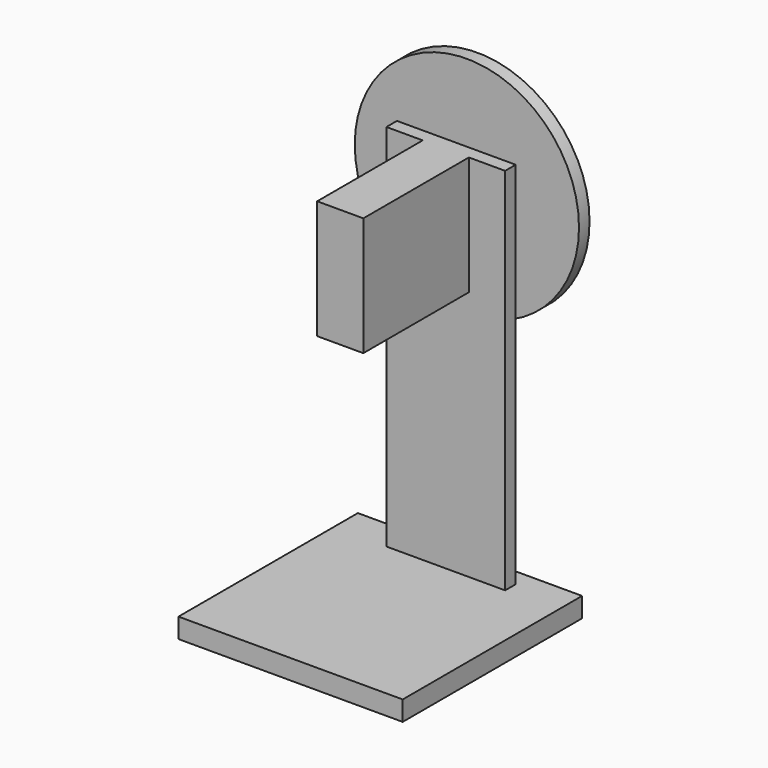
from build123d import *

# Parameters (mm, degrees)
F0_W      = 215.9
F0_H      = 215.9
F1_DEPTH  = 19.05
F3_W      = 114.3
F3_H      = 12.7
F4_DEPTH  = 355.6
F5_W      = 44.45
F5_H      = 127
F6_DEPTH  = 114.3
F9_R      = 6.35
F10_DEPTH = 12.7
F11_R     = 107.95
F12_DEPTH = 12.7


# Not quite as in the source:
# - a feature of the source that left no trace in its solid (it failed there, or was rolled back) is left out


with BuildPart() as f1:
    # F0 (on Top) → F1 (new body)
    with BuildSketch(Plane.XY):
        Rectangle(F0_W, F0_H)
    extrude(amount=F1_DEPTH)

    # F3 (on face) → F4 (join)
    with BuildSketch(Plane.XY.offset(19.05)):
        with Locations((0, 85.1799877524)):
            Rectangle(F3_W, F3_H)
    extrude(amount=F4_DEPTH)

    # F5 (on face) → F6 (join)
    with BuildSketch(Plane.XY.offset(374.65)):
        with Locations((0, 15.3299877524)):
            Rectangle(F5_W, F5_H)
    extrude(amount=-F6_DEPTH)

    # F9 (on face) → F10 (join)
    with BuildSketch(Plane(origin=(0, 91.5299877524, 0), x_dir=(-1, 0, 0), z_dir=(0, 1, 0))):
        with Locations((0, 332.823485136)):
            Circle(F9_R)
    extrude(amount=F10_DEPTH)

    # F11 (on face) → F12 (join)
    with BuildSketch(Plane(origin=(0, 104.2299877524, 0), x_dir=(-1, 0, 0), z_dir=(0, 1, 0))):
        with Locations((0, 332.823485136)):
            Circle(F11_R)
    extrude(amount=F12_DEPTH)


solid = f1.part
